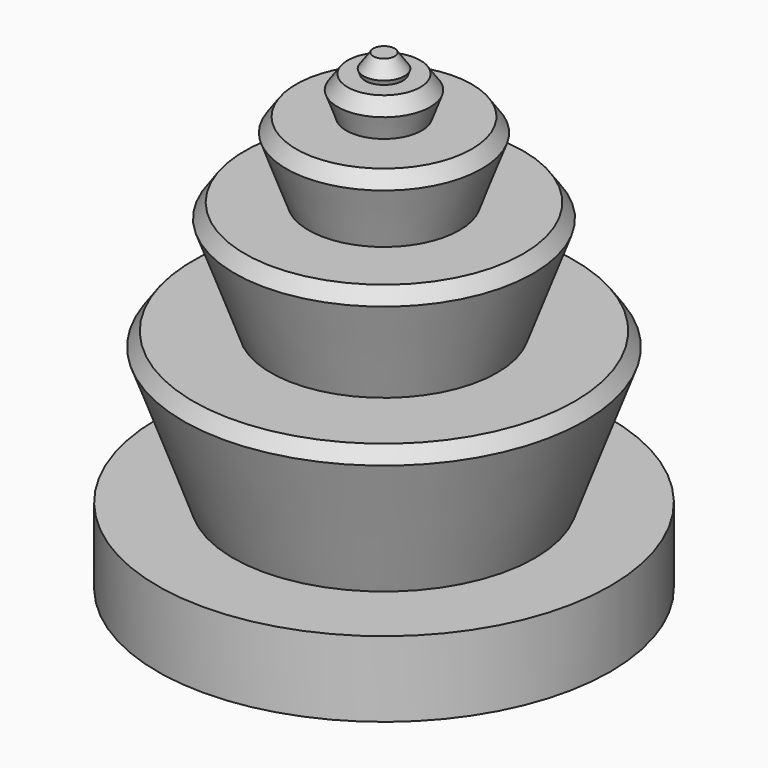
from build123d import *

# Parameters (mm, degrees)
F0_R      = 38.1
F1_DEPTH  = 12.7
F2_R      = 25.4
F3_DEPTH  = 25.4
F3_TAPER  = -20
F4_R      = 19.05
F5_DEPTH  = 19.05
F5_TAPER  = -20
F6_R      = 12.7
F7_DEPTH  = 12.7
F7_TAPER  = -20
F8_R      = 6.35
F9_DEPTH  = 6.35
F9_TAPER  = -20
F10_R     = 3.175
F11_DEPTH = 3.175
F11_TAPER = -20


# Not quite as in the source:
# - a fillet or chamfer that OpenCascade refuses, or shapes differently, is made with other operations: its cross-section is extruded or revolved along the edge and cut away or added


with BuildPart() as f1:
    # F0 (on Top) → F1 (new body)
    with BuildSketch(Plane.XY):
        Circle(F0_R)
    extrude(amount=F1_DEPTH)

    # F2 (on face) → F3 (join)
    with BuildSketch(Plane.XY.offset(12.7)):
        Circle(F2_R)
    extrude(amount=F3_DEPTH, taper=F3_TAPER)

    # F4 (on face) → F5 (join)
    with BuildSketch(Plane.XY.offset(38.1)):
        Circle(F4_R)
    extrude(amount=F5_DEPTH, taper=F5_TAPER)

    # F6 (on face) → F7 (join)
    with BuildSketch(Plane.XY.offset(57.15)):
        Circle(F6_R)
    extrude(amount=F7_DEPTH, taper=F7_TAPER)

    # F8 (on face) → F9 (join)
    with BuildSketch(Plane.XY.offset(69.85)):
        Circle(F8_R)
    extrude(amount=F9_DEPTH, taper=F9_TAPER)

    # F10 (on face) → F11 (join)
    with BuildSketch(Plane.XY.offset(76.2)):
        Circle(F10_R)
    extrude(amount=F11_DEPTH, taper=F11_TAPER)

    # F12: chamfer of 2.54 on 5 edges, made by hand

    # F12_s1 → F12_t2 (revolve, cut)
    with BuildSketch(Plane.XZ):
        Polygon((33.7761127863, 35.7131807432), (32.1048439504, 38.1), (34.6448439504, 38.1), align=None)
    revolve(axis=Axis((0, 0, 38.1), (0, 0, -1)), mode=Mode.SUBTRACT)

    # F12_s3 → F12_t4 (revolve, cut)
    with BuildSketch(Plane.XZ):
        Polygon((25.1149017987, 54.7631807432), (23.4436329628, 57.15), (25.9836329628, 57.15), align=None)
    revolve(axis=Axis((0, 0, 57.15), (0, 0, -1)), mode=Mode.SUBTRACT)

    # F12_s5 → F12_t6 (revolve, cut)
    with BuildSketch(Plane.XZ):
        Polygon((16.4536908111, 67.4631807432), (14.7824219752, 69.85), (17.3224219752, 69.85), align=None)
    revolve(axis=Axis((0, 0, 69.85), (0, 0, -1)), mode=Mode.SUBTRACT)

    # F12_s7 → F12_t8 (revolve, cut)
    with BuildSketch(Plane.XZ):
        Polygon((7.7924798235, 73.8131807432), (6.1212109876, 76.2), (8.6612109876, 76.2), align=None)
    revolve(axis=Axis((0, 0, 76.2), (0, 0, -1)), mode=Mode.SUBTRACT)

    # F12_s9 → F12_t10 (revolve, cut)
    with BuildSketch(Plane.XZ):
        Polygon((3.4618743297, 76.9881807432), (1.7906054938, 79.375), (4.3306054938, 79.375), align=None)
    revolve(axis=Axis((0, 0, 79.375), (0, 0, -1)), mode=Mode.SUBTRACT)


solid = f1.part
